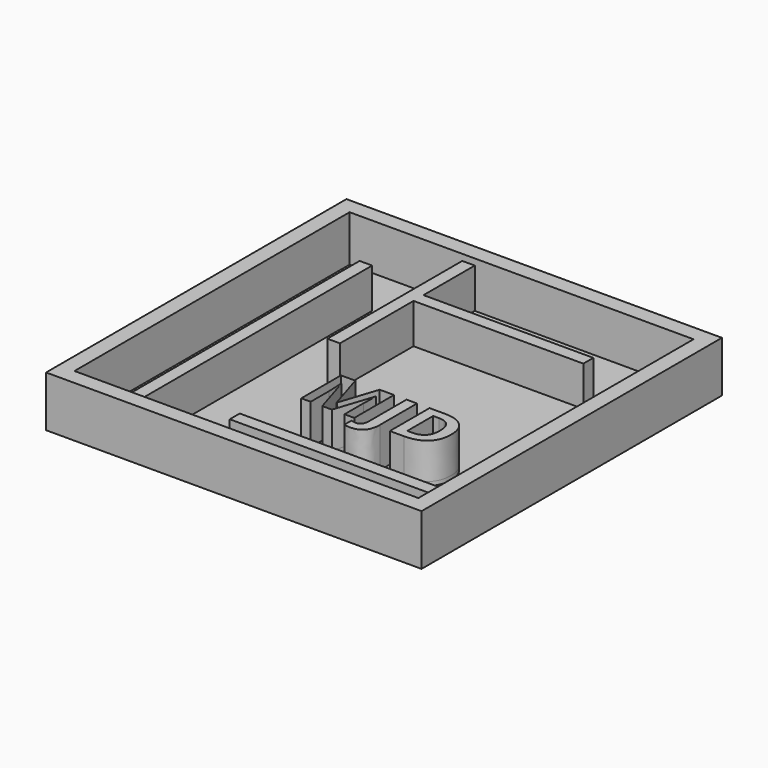
from build123d import *

# Parameters (mm, degrees)
F0_W         = 38.1
F0_H         = 38.1
F1_DEPTH     = 0.079375
F2_W         = 38.1
F2_H         = 38.1
F2_W_2       = 34.8996
F2_H_2       = 34.8996
F3_DEPTH     = 5.08
F4_W         = 1.27
F4_H         = 29.8196
F4_W_2       = 20.8812533696
F4_H_2       = 1.27
F5_DEPTH     = 4.445
F4_TEXT_SIZE = 7.0555555556
F6_DEPTH     = 4.445
F7_R         = 1.27
F8_DEPTH     = 0.79375
F9_DEPTH     = 0.396875


# Not quite as in the source:
# - Text() gives the source's letters only with a copy of the font that has no kerning and outlines rounded to 1/6400 em; it was checked with that copy


with BuildPart() as f1:
    # F0 (on Top) → F1 (new body)
    with BuildSketch(Plane.XY):
        with Locations((-3.6783535033, 3.1187085067)):
            Rectangle(F0_W, F0_H)
    extrude(amount=F1_DEPTH)

    # F2 (on face) → F3 (join)
    with BuildSketch(Plane.XY.offset(0.079375)):
        with Locations((-3.6783535033, 3.1187085067)):
            Rectangle(F2_W, F2_H)
        with Locations((-3.6783535033, 3.1187085067)):
            Rectangle(F2_W_2, F2_H_2, mode=Mode.SUBTRACT)
    extrude(amount=F3_DEPTH)

    # F4 (on face) → F5 (join)
    with BuildSketch(Plane.XY.offset(0.079375)):
        with Locations((-15.4131535033, 0.5787085067)):
            Rectangle(F4_W, F4_H)
        Polygon((-8.4281535033, 20.5685085067), (-9.6981535033, 20.5685085067), (-9.6981535033, 3.4687234357), (-8.4281535033, 3.4687234357), (-8.4281535033, 12.798121199), (8.8063962758, 12.798121199), (8.8063962758, 14.068121199), (-8.4281535033, 14.068121199), align=None)
        with Locations((3.3308198119, -11.5241848464)):
            Rectangle(F4_W_2, F4_H_2)
    extrude(amount=F5_DEPTH)

    # F4 (on face) → F6 (join)
    with BuildSketch(Plane.XY.offset(0.079375)):
        with Locations((-15.4131535033, 0.5787085067)):
            Rectangle(F4_W, F4_H)
        with Locations((3.3308198119, -11.5241848464)):
            Rectangle(F4_W_2, F4_H_2)
        Polygon((-8.4281535033, 14.068121199), (-8.4281535033, 20.5685085067), (-9.6981535033, 20.5685085067), (-9.6981535033, 3.4687234357), (-8.4281535033, 3.4687234357), (-8.4281535033, 12.798121199), (8.8063962758, 12.798121199), (8.8063962758, 14.068121199), align=None)
        with Locations((-5.5673903089, -5.8091848464)):
            Text('MJD', F4_TEXT_SIZE, font='Open Sans', font_style=FontStyle.BOLD, text_align=(TextAlign.LEFT, TextAlign.BOTTOM))
    extrude(amount=F6_DEPTH)

    # F7 (on face) → F8 (join)
    with BuildSketch(Plane.XY.offset(0.079375)):
        Polygon((-21.1281535033, 20.5685085067), (-21.1281535033, -14.3310914933), (-16.0481535033, -14.3310914933), (-16.0481535033, 15.4885085067), (-14.7781535033, 15.4885085067), (-14.7781535033, -14.3310914933), (13.7714464967, -14.3310914933), (13.7714464967, -12.1591848464), (-7.1098068729, -12.1591848464), (-7.1098068729, -10.8891848464), (13.7714464967, -10.8891848464), (13.7714464967, 20.5685085067), (-8.4281535033, 20.5685085067), (-8.4281535033, 14.068121199), (8.8063962758, 14.068121199), (8.8063962758, 12.798121199), (-8.4281535033, 12.798121199), (-8.4281535033, 3.4687234357), (-9.6981535033, 3.4687234357), (-9.6981535033, 20.5685085067), (-11.9173903089, 20.5685085067), align=None)
        with Locations((-18.7506005168, -10.1872691885)):
            Circle(F7_R, mode=Mode.SUBTRACT)
        with BuildLine():
            Line((-0.5237705172, -1.8646883187), (-1.8224337117, -5.8091848464))
            Line((-1.8224337117, -5.8091848464), (-2.801392045, -5.8091848464))
            Line((-2.801392045, -5.8091848464), (-4.0140656561, -1.8580737353))
            Line((-4.0140656561, -1.8580737353), (-4.0449337117, -1.8580737353))
            add(Edge.make_bspline(
                [(-4.0449337117, -1.8580737353), (-3.9787878783, -3.0630303325), (-3.9787878783, -3.4665199159)],
                knots=[0, 0, 0, 1, 1, 1], degree=2))
            Line((-3.9787878783, -3.4665199159), (-3.9787878783, -5.8091848464))
            Line((-3.9787878783, -5.8091848464), (-4.9334927395, -5.8091848464))
            Line((-4.9334927395, -5.8091848464), (-4.9334927395, -0.7721796381))
            Line((-4.9334927395, -0.7721796381), (-3.4793868367, -0.7721796381))
            Line((-3.4793868367, -0.7721796381), (-2.2876594061, -4.6240719992))
            Line((-2.2876594061, -4.6240719992), (-2.2667132256, -4.6240719992))
            Line((-2.2667132256, -4.6240719992), (-1.0022253783, -0.7721796381))
            Line((-1.0022253783, -0.7721796381), (0.4507780939, -0.7721796381))
            Line((0.4507780939, -0.7721796381), (0.4507780939, -5.8091848464))
            Line((0.4507780939, -5.8091848464), (-0.5447166978, -5.8091848464))
            Line((-0.5447166978, -5.8091848464), (-0.5447166978, -3.4246275548))
            add(Edge.make_bspline(
                [(-0.5447166978, -3.4246275548), (-0.5447166978, -3.2559556798), (-0.539204545, -3.0354695687)],
                knots=[0, 0, 0, 1, 1, 1], degree=2))
            add(Edge.make_bspline(
                [(-0.539204545, -3.0354695687), (-0.5336923922, -2.8149834575), (-0.4929024617, -1.8646883187)],
                knots=[0, 0, 0, 1, 1, 1], degree=2))
            Line((-0.4929024617, -1.8646883187), (-0.5237705172, -1.8646883187))
        make_face(mode=Mode.SUBTRACT)
        with BuildLine():
            add(Edge.make_bspline(
                [(2.7868284411, -5.4850702631), (2.7868284411, -6.3670147075), (2.383890073, -6.8289331103)],
                knots=[0, 0, 0, 1, 1, 1], degree=2))
            add(Edge.make_bspline(
                [(2.383890073, -6.8289331103), (1.980951705, -7.2908515131), (1.1916114272, -7.2908515131)],
                knots=[0, 0, 0, 1, 1, 1], degree=2))
            add(Edge.make_bspline(
                [(1.1916114272, -7.2908515131), (0.830014205, -7.2908515131), (0.5610211494, -7.2147838048)],
                knots=[0, 0, 0, 1, 1, 1], degree=2))
            Line((0.5610211494, -7.2147838048), (0.5610211494, -6.326224777))
            add(Edge.make_bspline(
                [(0.5610211494, -6.326224777), (0.8366287883, -6.3945754714), (1.0637294828, -6.3945754714)],
                knots=[0, 0, 0, 1, 1, 1], degree=2))
            add(Edge.make_bspline(
                [(1.0637294828, -6.3945754714), (1.41540483, -6.3945754714), (1.5669890314, -6.1757430062)],
                knots=[0, 0, 0, 1, 1, 1], degree=2))
            add(Edge.make_bspline(
                [(1.5669890314, -6.1757430062), (1.7185732328, -5.9569105409), (1.7185732328, -5.4916848464)],
                knots=[0, 0, 0, 1, 1, 1], degree=2))
            Line((1.7185732328, -5.4916848464), (1.7185732328, -0.7721796381))
            Line((1.7185732328, -0.7721796381), (2.7868284411, -0.7721796381))
            Line((2.7868284411, -0.7721796381), (2.7868284411, -5.4850702631))
        make_face(mode=Mode.SUBTRACT)
        with BuildLine():
            add(Edge.make_bspline(
                [(5.6355089967, -0.7721796381), (6.8691287883, -0.7721796381), (7.5515333022, -1.4231648812)],
                knots=[0, 0, 0, 1, 1, 1], degree=2))
            add(Edge.make_bspline(
                [(7.5515333022, -1.4231648812), (8.2339378161, -2.0741501242), (8.2339378161, -3.2427265131)],
                knots=[0, 0, 0, 1, 1, 1], degree=2))
            add(Edge.make_bspline(
                [(8.2339378161, -3.2427265131), (8.2339378161, -4.4862681798), (7.5256261842, -5.1477265131)],
                knots=[0, 0, 0, 1, 1, 1], degree=2))
            add(Edge.make_bspline(
                [(7.5256261842, -5.1477265131), (6.8173145522, -5.8091848464), (5.4811687189, -5.8091848464)],
                knots=[0, 0, 0, 1, 1, 1], degree=2))
            Line((5.4811687189, -5.8091848464), (4.05462358, -5.8091848464))
            Line((4.05462358, -5.8091848464), (4.05462358, -0.7721796381))
            Line((4.05462358, -0.7721796381), (5.6355089967, -0.7721796381))
        make_face(mode=Mode.SUBTRACT)
        with Locations((-5.0040357746, 17.1852447093)):
            Circle(F7_R, mode=Mode.SUBTRACT)
    extrude(amount=F8_DEPTH)

    # F9 (cut): a face of the model
    f9_faces = [f1.faces().sort_by_distance(p)[0] for p in [
        (-3.5602976096, 3.4486000721, 0.873125),
    ]]
    extrude(f9_faces, amount=-F9_DEPTH, mode=Mode.SUBTRACT)


solid = f1.part
